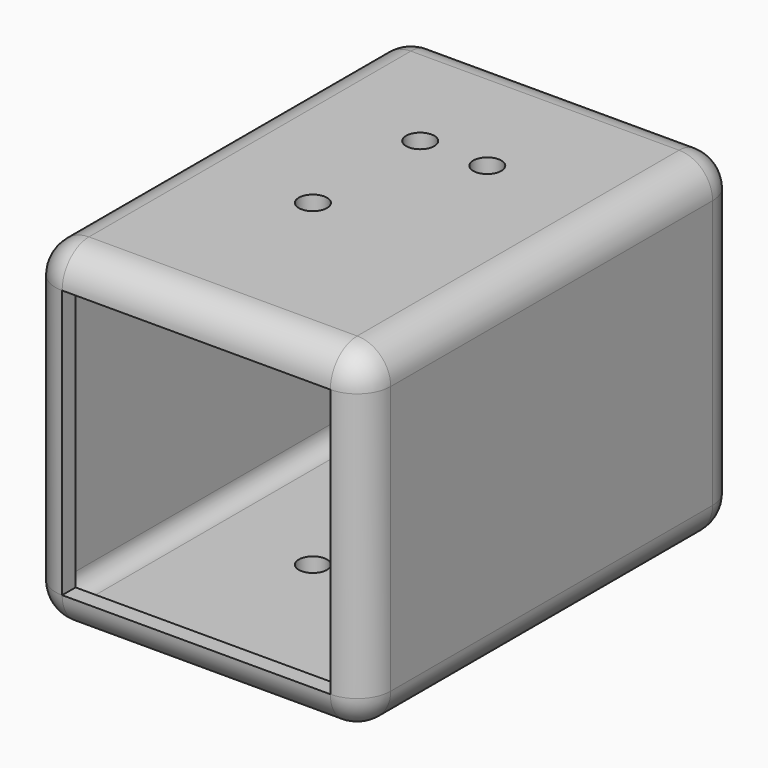
from build123d import *

# Parameters (mm, degrees)
F1_DEPTH = 35
F2_R     = 5
F3_T     = -2.5
F5_D     = 4.2


# Not quite as in the source:
# - a shell that OpenCascade refuses in one call is made with other operations: the cavity is built on its own and cut out


with BuildPart() as f1:
    # F0 (on Front) → F1 (new body, symmetric)
    with BuildSketch(Plane.XZ):
        with BuildLine():
            Line((20, 25), (-20, 25))
            ThreePointArc((-20, 25), (-23.5355339059, 23.5355339059), (-25, 20))
            Line((-25, 20), (-25, -20))
            ThreePointArc((-25, -20), (-23.5355339059, -23.5355339059), (-20, -25))
            Line((-20, -25), (20, -25))
            ThreePointArc((20, -25), (23.5355339059, -23.5355339059), (25, -20))
            Line((25, -20), (25, 20))
            ThreePointArc((25, 20), (23.5355339059, 23.5355339059), (20, 25))
        make_face()
    extrude(amount=F1_DEPTH, both=True)

    # F2
    f2_edges = [f1.edges().sort_by_distance(p)[0] for p in [
        (0, 35, 25),
        (-23.535534, 35, 23.535534),
        (-25, 35, 0),
        (-23.535534, 35, -23.535534),
        (0, 35, -25),
        (23.535534, 35, -23.535534),
        (25, 35, 0),
        (23.535534, 35, 23.535534),
        (0, -35, 25),
        (-23.535534, -35, 23.535534),
        (-25, -35, 0),
        (-23.535534, -35, -23.535534),
        (0, -35, -25),
        (23.535534, -35, -23.535534),
        (25, -35, 0),
        (23.535534, -35, 23.535534),
    ]]
    fillet(f2_edges, radius=F2_R)

    # F3: a shell. OpenCascade refuses it in one call, so the cavity is built on its own and cut out:
    # the body offset inwards by the wall thickness, plus a prism from it out through each open face.
    f3_core = offset(f1.part, amount=F3_T, mode=Mode.PRIVATE)
    f3_exits = [f3_core.faces().sort_by_distance(p)[0] for p in [
        (0, -32.5, 0),
    ]]
    add(f3_core, mode=Mode.SUBTRACT)
    extrude(f3_exits, amount=-F3_T, mode=Mode.SUBTRACT)

    # F5 (through all)
    with Locations(Plane(origin=(0, 0, -25), x_dir=(1, 0, 0), z_dir=(0, 0, -1))):
        with Locations((5, -13), (-5, 7), (-5, -13)):
            Hole(F5_D / 2)


solid = f1.part
